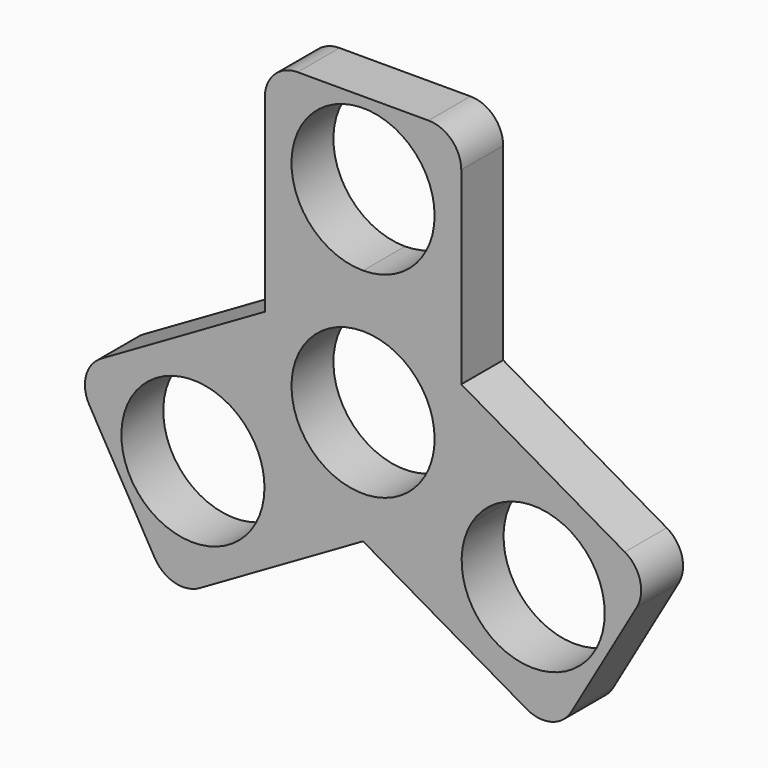
from build123d import *

# Parameters (mm, degrees)
F1_DEPTH = 8


with BuildPart() as f1:
    # F0 (on Front) → F1 (new body)
    with BuildSketch(Plane.XZ):
        with BuildLine():
            Line((-182.0272845483, 7.2368355937), (-178.701967001, 5.3169626126))
            Line((-178.701967001, 5.3169626126), (-175.3766494537, 7.2368355937))
            Line((-175.3766494537, 7.2368355937), (-172.0513319064, 1.4772166504))
            Line((-172.0513319064, 1.4772166504), (-163.701967001, -3.3432914252))
            Line((-163.701967001, -3.3432914252), (-163.701967001, 25.4964545369))
            ThreePointArc((-163.701967001, 25.4964545369), (-165.166433095, 29.0319884428), (-168.701967001, 30.4964545369))
            Line((-168.701967001, 30.4964545369), (-188.701967001, 30.4964545369))
            ThreePointArc((-188.701967001, 30.4964545369), (-192.2375009069, 29.0319884428), (-193.701967001, 25.4964545369))
            Line((-193.701967001, 25.4964545369), (-193.701967001, -3.3432914252))
            Line((-193.701967001, -3.3432914252), (-185.3526020956, 1.4772166504))
            Line((-185.3526020956, 1.4772166504), (-182.0272845483, 7.2368355937))
        make_face()
        with BuildLine():
            ThreePointArc((-167.776967001, 17.9964545369), (-170.9768254165, 10.2713129525), (-178.701967001, 7.0714545369))
            ThreePointArc((-178.701967001, 7.0714545369), (-186.4271085854, 25.7215961214), (-167.776967001, 17.9964545369))
        make_face(mode=Mode.SUBTRACT)
        with BuildLine():
            Line((-160.3766494537, -18.7439265199), (-163.701967001, -20.6637995009))
            Line((-163.701967001, -20.6637995009), (-163.701967001, -24.5035454631))
            Line((-163.701967001, -24.5035454631), (-170.3526020956, -24.5035454631))
            Line((-170.3526020956, -24.5035454631), (-178.701967001, -29.3240535388))
            Line((-178.701967001, -29.3240535388), (-153.726014359, -43.7439265199))
            ThreePointArc((-153.726014359, -43.7439265199), (-149.9319191335, -44.2434286324), (-146.8958873401, -41.9137995009))
            Line((-146.8958873401, -41.9137995009), (-136.8958873401, -24.5932914252))
            ThreePointArc((-136.8958873401, -24.5932914252), (-136.3963852276, -20.7991961997), (-138.726014359, -17.7631644063))
            Line((-138.726014359, -17.7631644063), (-163.701967001, -3.3432914252))
            Line((-163.701967001, -3.3432914252), (-163.701967001, -12.9843075766))
            Line((-163.701967001, -12.9843075766), (-160.3766494537, -18.7439265199))
        make_face()
        with BuildLine():
            ThreePointArc((-141.7962048874, -27.0035454631), (-155.5488029552, -37.5562851153), (-162.1825324238, -21.5410454631))
            ThreePointArc((-162.1825324238, -21.5410454631), (-149.8936068197, -16.4508058109), (-141.7962048874, -27.0035454631))
        make_face(mode=Mode.SUBTRACT)
        with BuildLine():
            Line((-193.701967001, -24.5035454631), (-193.701967001, -20.6637995009))
            Line((-193.701967001, -20.6637995009), (-197.0272845483, -18.7439265199))
            Line((-197.0272845483, -18.7439265199), (-193.701967001, -12.9843075766))
            Line((-193.701967001, -12.9843075766), (-193.701967001, -3.3432914252))
            Line((-193.701967001, -3.3432914252), (-218.6779196429, -17.7631644063))
            ThreePointArc((-218.6779196429, -17.7631644063), (-221.0075487743, -20.7991961997), (-220.5080466618, -24.5932914252))
            Line((-220.5080466618, -24.5932914252), (-210.5080466618, -41.9137995009))
            ThreePointArc((-210.5080466618, -41.9137995009), (-207.4720148684, -44.2434286324), (-203.6779196429, -43.7439265199))
            Line((-203.6779196429, -43.7439265199), (-178.701967001, -29.3240535388))
            Line((-178.701967001, -29.3240535388), (-187.0513319064, -24.5035454631))
            Line((-187.0513319064, -24.5035454631), (-193.701967001, -24.5035454631))
        make_face()
        with BuildLine():
            ThreePointArc((-193.7577291145, -27.0035454631), (-215.2354687667, -29.8311435308), (-195.2214015781, -21.5410454631))
            ThreePointArc((-195.2214015781, -21.5410454631), (-194.1299894623, -24.1759473953), (-193.7577291145, -27.0035454631))
        make_face(mode=Mode.SUBTRACT)
        Polygon((-193.701967001, -12.9843075766), (-185.3526020956, 1.4772166504), (-193.701967001, -3.3432914252), align=None)
        Polygon((-163.701967001, -3.3432914252), (-172.0513319064, 1.4772166504), (-163.701967001, -12.9843075766), align=None)
        Polygon((-178.701967001, -29.3240535388), (-170.3526020956, -24.5035454631), (-187.0513319064, -24.5035454631), align=None)
        with BuildLine():
            ThreePointArc((-188.1632945373, -17.4660454631), (-188.1632945373, -6.5410454631), (-178.701967001, -1.0785454631))
            Line((-178.701967001, -1.0785454631), (-178.701967001, 5.3169626126))
            Line((-178.701967001, 5.3169626126), (-185.3526020956, 1.4772166504))
            Line((-185.3526020956, 1.4772166504), (-193.701967001, -12.9843075766))
            Line((-193.701967001, -12.9843075766), (-193.701967001, -20.6637995009))
            Line((-193.701967001, -20.6637995009), (-188.1632945373, -17.4660454631))
        make_face()
        with BuildLine():
            ThreePointArc((-178.701967001, -1.0785454631), (-170.9768254165, -4.2784038786), (-167.776967001, -12.0035454631))
            ThreePointArc((-167.776967001, -12.0035454631), (-168.1492273488, -14.8311435308), (-169.2406394646, -17.4660454631))
            Line((-169.2406394646, -17.4660454631), (-163.701967001, -20.6637995009))
            Line((-163.701967001, -20.6637995009), (-163.701967001, -12.9843075766))
            Line((-163.701967001, -12.9843075766), (-172.0513319064, 1.4772166504))
            Line((-172.0513319064, 1.4772166504), (-178.701967001, 5.3169626126))
            Line((-178.701967001, 5.3169626126), (-178.701967001, -1.0785454631))
        make_face()
        Polygon((-175.3766494537, 7.2368355937), (-178.701967001, 5.3169626126), (-172.0513319064, 1.4772166504), align=None)
        Polygon((-185.3526020956, 1.4772166504), (-178.701967001, 5.3169626126), (-182.0272845483, 7.2368355937), align=None)
        with BuildLine():
            Line((-163.701967001, -20.6637995009), (-169.2406394646, -17.4660454631))
            ThreePointArc((-169.2406394646, -17.4660454631), (-178.701967001, -22.9285454631), (-188.1632945373, -17.4660454631))
            Line((-188.1632945373, -17.4660454631), (-193.701967001, -20.6637995009))
            Line((-193.701967001, -20.6637995009), (-187.0513319064, -24.5035454631))
            Line((-187.0513319064, -24.5035454631), (-170.3526020956, -24.5035454631))
            Line((-170.3526020956, -24.5035454631), (-163.701967001, -20.6637995009))
        make_face()
        Polygon((-163.701967001, -12.9843075766), (-163.701967001, -20.6637995009), (-160.3766494537, -18.7439265199), align=None)
        Polygon((-163.701967001, -24.5035454631), (-163.701967001, -20.6637995009), (-170.3526020956, -24.5035454631), align=None)
        Polygon((-187.0513319064, -24.5035454631), (-193.701967001, -20.6637995009), (-193.701967001, -24.5035454631), align=None)
        Polygon((-197.0272845483, -18.7439265199), (-193.701967001, -20.6637995009), (-193.701967001, -12.9843075766), align=None)
    extrude(amount=F1_DEPTH)


solid = f1.part
